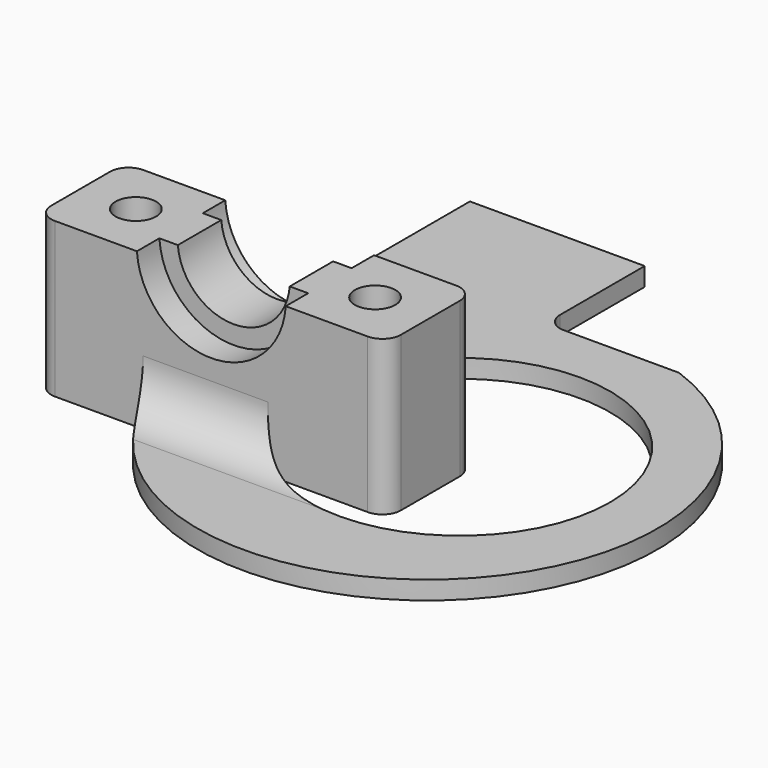
from build123d import *

# Parameters (mm, degrees)
F0_W          = 38
F0_H          = 12
F0_R          = 2.2
F1_DEPTH      = 16.8
F3_DEPTH      = 12.001
F4_R          = 8.1
F5_DEPTH      = 3.05
F6_R          = 8.1
F7_DEPTH      = 3.05
F8_R          = 16.345
F9_DEPTH      = 2
F10_R         = 1.45
F11_DEPTH     = 16.801
F12_R         = 4.5
F12_R_2       = 2.2
F13_DEPTH     = 9
F14_SIZE      = 2.29999
F15_T4_DEPTH  = 23.6674466009
F15_S5_R      = 16.345
F15_T6_DEPTH  = 14
F15_S7_R      = 1.45
F15_T8_DEPTH  = 14
F15_T12_DEPTH = 38.54569481
F15_S13_R     = 25
F15_T14_DEPTH = 21
F15_S15_R     = 16.345
F15_T16_DEPTH = 21
F16_T1_DEPTH  = 2
F16_T3_DEPTH  = 26.8


# Not quite as in the source:
# - a fillet or chamfer that OpenCascade refuses, or shapes differently, is made with other operations: its cross-section is extruded or revolved along the edge and cut away or added
# - a fillet or chamfer is up to 0.001 mm smaller than in the source, because OpenCascade refuses the exact size


with BuildPart() as f1:
    # F0 (on Top) → F1 (new body)
    with BuildSketch(Plane.XY):
        Rectangle(F0_W, F0_H)
        with Locations((-13, 0)):
            Circle(F0_R, mode=Mode.SUBTRACT)
        with Locations((13, 0)):
            Circle(F0_R, mode=Mode.SUBTRACT)
    extrude(amount=F1_DEPTH)

    # F2 (on face) → F3 (cut, through all)
    with BuildSketch(Plane(origin=(0, 6, 0), x_dir=(-1, 0, 0), z_dir=(0, 1, 0))):
        with BuildLine():
            ThreePointArc((-6.0794736614, 16.8), (0, 11.2), (6.0794736614, 16.8))
            Line((6.0794736614, 16.8), (-6.0794736614, 16.8))
        make_face()
        with BuildLine():
            Line((-6.0794736614, 16.8), (6.0794736614, 16.8))
            ThreePointArc((6.0794736614, 16.8), (6.0948662551, 17.0497894234), (6.1, 17.3))
            ThreePointArc((6.1, 17.3), (-0.2502105766, 23.3948662551), (-6.0794736614, 16.8))
        make_face()
    extrude(amount=-F3_DEPTH, mode=Mode.SUBTRACT)

    # F4 (on face) → F5 (cut)
    with BuildSketch(Plane(origin=(0, 6, 0), x_dir=(-1, 0, 0), z_dir=(0, 1, 0))):
        with Locations((0, 17.3)):
            Circle(F4_R)
    extrude(amount=-F5_DEPTH, mode=Mode.SUBTRACT)

    # F6 (on face) → F7 (cut)
    with BuildSketch(Plane.XZ.offset(6)):
        with Locations((0, 17.3)):
            Circle(F6_R)
    extrude(amount=-F7_DEPTH, mode=Mode.SUBTRACT)

    # F8 (on Top) → F9 (join)
    with BuildSketch(Plane.XY):
        with BuildLine():
            Line((-9.5, 41), (-9.5, 4))
            ThreePointArc((-9.5, 4), (29.848439809, -16.4722441189), (24.03, 27.5))
            Line((24.03, 27.5), (9.5, 27.5))
            Line((9.5, 27.5), (9.5, 41))
            Line((9.5, 41), (-9.5, 41))
        make_face()
        with Locations((17.995, 5.245)):
            Circle(F8_R, mode=Mode.SUBTRACT)
    extrude(amount=F9_DEPTH)

    # F10 (on face) → F11 (cut, through all)
    with BuildSketch(Plane(origin=(0, 0, 0), x_dir=(1, 0, 0), z_dir=(0, 0, -1))):
        with Locations((-5, -10.5)):
            Circle(F10_R)
        with Locations((-5, -25.5)):
            Circle(F10_R)
    extrude(amount=-F11_DEPTH, mode=Mode.SUBTRACT)

    # F12 (on face) → F13 (cut)
    with BuildSketch(Plane(origin=(0, 0, 0), x_dir=(1, 0, 0), z_dir=(0, 0, -1))):
        with Locations((-13, 0)):
            Circle(F12_R)
        with Locations((-13, 0)):
            Circle(F12_R_2, mode=Mode.SUBTRACT)
        with Locations((13, 0)):
            Circle(F12_R)
        with Locations((13, 0)):
            Circle(F12_R_2, mode=Mode.SUBTRACT)
    extrude(amount=-F13_DEPTH, mode=Mode.SUBTRACT)

    # F14 (size 2.3 in the source; OpenCascade refuses exactly that, so slightly less here)
    f14_edges = [f1.edges().sort_by_distance(p)[0] for p in [
        (-17.5, 0, 9),
        (8.5, 0, 9),
    ]]
    chamfer(f14_edges, length=F14_SIZE)

    # F15: fillet of radius 5 on 2 edges, made by hand


with BuildPart() as f15_tool2:
    # F15_s3 → F15_t4 (new body)
    with BuildSketch(Plane.YZ.offset(14.1674466009)):
        with BuildLine():
            ThreePointArc((6, 7), (7.4644660941, 3.4644660941), (11, 2))
            Line((11, 2), (6, 2))
            Line((6, 2), (6, 7))
        make_face()
    extrude(amount=-F15_T4_DEPTH)

    # F15_s5 → F15_t6 (cut, symmetric)
    with BuildSketch(Plane.XY.offset(4.5)):
        with Locations((17.995, 5.245)):
            Circle(F15_S5_R)
    extrude(amount=F15_T6_DEPTH, both=True, mode=Mode.SUBTRACT)

    # F15_s7 → F15_t8 (cut, symmetric)
    with BuildSketch(Plane.XY.offset(4.5)):
        with Locations((-5, 10.5)):
            Circle(F15_S7_R)
    extrude(amount=F15_T8_DEPTH, both=True, mode=Mode.SUBTRACT)


with BuildPart() as f1_1:
    add(f1.part)

    # F15_t1: union F15_tool2
    add(f15_tool2.part)


with BuildPart() as f15_tool10:
    # F15_s11 → F15_t12 (new body)
    with BuildSketch(Plane.YZ.offset(-19.9127772578)):
        with BuildLine():
            ThreePointArc((-6, 7), (-7.4644660941, 3.4644660941), (-11, 2))
            Line((-11, 2), (-6, 2))
            Line((-6, 2), (-6, 7))
        make_face()
    extrude(amount=F15_T12_DEPTH)

    # F15_s13 → F15_t14 (intersect, symmetric)
    with BuildSketch(Plane.XY.offset(4.5)):
        with Locations((15.4999999989, 4.0002319164)):
            Circle(F15_S13_R)
    extrude(amount=F15_T14_DEPTH, both=True, mode=Mode.INTERSECT)

    # F15_s15 → F15_t16 (cut, symmetric)
    with BuildSketch(Plane.XY.offset(4.5)):
        with Locations((17.995, 5.245)):
            Circle(F15_S15_R)
    extrude(amount=F15_T16_DEPTH, both=True, mode=Mode.SUBTRACT)


with BuildPart() as f1_2:
    add(f1_1.part)

    # F15_t9: union F15_tool10
    add(f15_tool10.part)

    # F16: fillet of radius 2 on 5 edges, made by hand

    # F16_s2 → F16_t1 (join)
    with BuildSketch(Plane.XY):
        with BuildLine():
            ThreePointArc((9.5, 29.5), (10.0857864376, 28.0857864376), (11.5, 27.5))
            Line((11.5, 27.5), (9.5, 27.5))
            Line((9.5, 27.5), (9.5, 29.5))
        make_face()
    extrude(amount=F16_T1_DEPTH)

    # F16_s4 → F16_t3 (cut)
    with BuildSketch(Plane.XY.offset(-5)):
        with BuildLine():
            ThreePointArc((17, 6), (18.4142135624, 5.4142135624), (19, 4))
            Line((19, 4), (19, 6))
            Line((19, 6), (17, 6))
        make_face()
        with BuildLine():
            ThreePointArc((17, -6), (18.4142135624, -5.4142135624), (19, -4))
            Line((19, -4), (19, -6))
            Line((19, -6), (17, -6))
        make_face()
        with BuildLine():
            ThreePointArc((-19, 4), (-18.4142135624, 5.4142135624), (-17, 6))
            Line((-17, 6), (-19, 6))
            Line((-19, 6), (-19, 4))
        make_face()
        with BuildLine():
            ThreePointArc((-17, -6), (-18.4142135624, -5.4142135624), (-19, -4))
            Line((-19, -4), (-19, -6))
            Line((-19, -6), (-17, -6))
        make_face()
    extrude(amount=F16_T3_DEPTH, mode=Mode.SUBTRACT)


solid = f1_2.part
